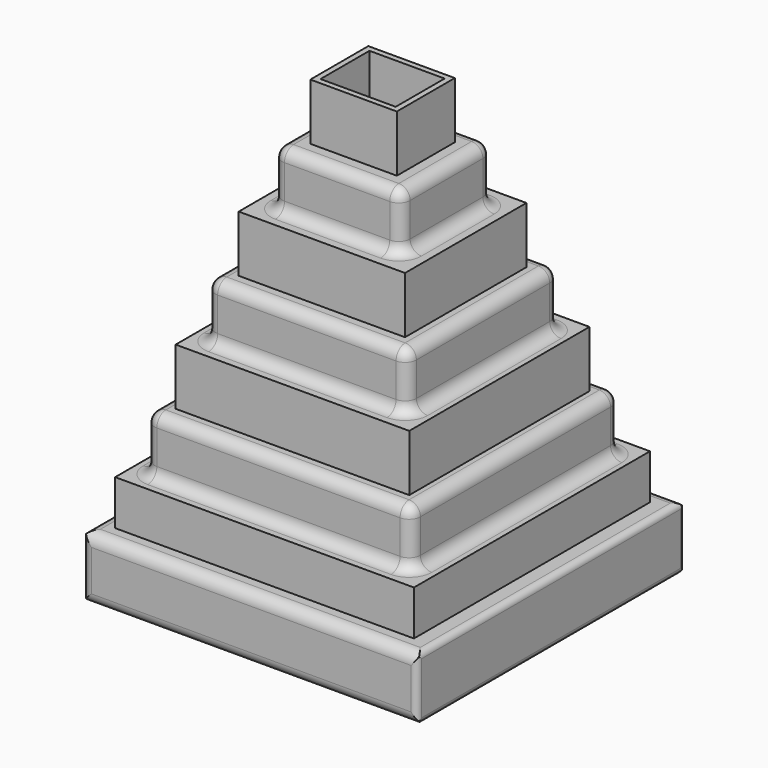
from build123d import *

# Parameters (mm, degrees)
F0_W         = 151.3316631317
F0_H         = 150.4956334829
F1_DEPTH     = 28.5412985831
F2_W         = 134.191930294
F2_H         = 132.5197666883
F3_DEPTH     = 20.1653186232
F4_W         = 119.4145902991
F4_H         = 116.9039234519
F5_DEPTH     = 25.4
F6_W         = 104.9288511276
F6_H         = 101.1665165424
F7_DEPTH     = 25.4
F8_W         = 90.2792215347
F8_H         = 84.9945694208
F9_DEPTH     = 25.4
F10_W        = 74.6954381466
F10_H        = 68.1595951319
F11_DEPTH    = 25.4
F12_W        = 57.4390292168
F12_H        = 51.001906395
F13_DEPTH    = 25.4
F14_W        = 38.8528704643
F14_H        = 32.552421093
F15_DEPTH    = 25.4
F16_T        = -2.54
F17_R        = 2.5998669894
F18_T1_DEPTH = 174.1317961423
F18_T3_DEPTH = 53.9412985831
F19_T1_DEPTH = 170.815633483
F19_T3_DEPTH = 53.9412985831
F20_T1_DEPTH = 169.0517961423
F21_R        = 5.08


# Not quite as in the source:
# - a fillet or chamfer that OpenCascade refuses, or shapes differently, is made with other operations: its cross-section is extruded or revolved along the edge and cut away or added


with BuildPart() as f1:
    # F0 (on Top) → F1 (new body)
    with BuildSketch(Plane.XY):
        Rectangle(F0_W, F0_H)
    extrude(amount=F1_DEPTH)

    # F2 (on face) → F3 (join)
    with BuildSketch(Plane.XY.offset(28.5412985831)):
        Rectangle(F2_W, F2_H)
    extrude(amount=F3_DEPTH)

    # F4 (on face) → F5 (join)
    with BuildSketch(Plane.XY.offset(48.7066172063)):
        Rectangle(F4_W, F4_H)
    extrude(amount=F5_DEPTH)

    # F6 (on face) → F7 (join)
    with BuildSketch(Plane.XY.offset(74.1066172063)):
        Rectangle(F6_W, F6_H)
    extrude(amount=F7_DEPTH)

    # F8 (on face) → F9 (join)
    with BuildSketch(Plane.XY.offset(99.5066172063)):
        Rectangle(F8_W, F8_H)
    extrude(amount=F9_DEPTH)

    # F10 (on face) → F11 (join)
    with BuildSketch(Plane.XY.offset(124.9066172063)):
        Rectangle(F10_W, F10_H)
    extrude(amount=F11_DEPTH)

    # F12 (on face) → F13 (join)
    with BuildSketch(Plane.XY.offset(150.3066172063)):
        Rectangle(F12_W, F12_H)
    extrude(amount=F13_DEPTH)

    # F14 (on face) → F15 (join)
    with BuildSketch(Plane.XY.offset(175.7066172063)):
        Rectangle(F14_W, F14_H)
    extrude(amount=F15_DEPTH)

    # F16
    f16_openings = [f1.faces().sort_by_distance(p)[0] for p in [
        (0, 0, 201.106617),
    ]]
    offset(amount=F16_T, openings=f16_openings, kind=Kind.INTERSECTION)

    # F17
    f17_edges = [f1.edges().sort_by_distance(p)[0] for p in [
        (75.665832, -75.247817, 14.270649),
        (75.665832, 75.247817, 14.270649),
        (75.665832, 0, 0),
        (75.665832, 0, 28.541299),
    ]]
    fillet(f17_edges, radius=F17_R)

    # F18: fillet of radius 5.08 on 4 edges, made by hand

    # F18_s2 → F18_t1 (cut)
    with BuildSketch(Plane.YZ.offset(-88.3658315659)):
        with BuildLine():
            ThreePointArc((-75.2478167415, 5.08), (-73.7599191899, 1.4878975516), (-70.1678167415, 0))
            Line((-70.1678167415, 0), (-75.2478167415, 0))
            Line((-75.2478167415, 0), (-75.2478167415, 5.08))
        make_face()
        with BuildLine():
            ThreePointArc((-75.2478167415, 23.4612985831), (-73.7599191899, 27.0534010316), (-70.1678167415, 28.5412985831))
            Line((-70.1678167415, 28.5412985831), (-75.2478167415, 28.5412985831))
            Line((-75.2478167415, 28.5412985831), (-75.2478167415, 23.4612985831))
        make_face()
    extrude(amount=F18_T1_DEPTH, mode=Mode.SUBTRACT)

    # F18_s4 → F18_t3 (cut)
    with BuildSketch(Plane.XY.offset(-12.7)):
        with BuildLine():
            ThreePointArc((-70.5858315659, -75.2478167415), (-74.1779340143, -73.7599191899), (-75.6658315659, -70.1678167415))
            Line((-75.6658315659, -70.1678167415), (-75.6658315659, -75.2478167415))
            Line((-75.6658315659, -75.2478167415), (-70.5858315659, -75.2478167415))
        make_face()
    extrude(amount=F18_T3_DEPTH, mode=Mode.SUBTRACT)

    # F19: fillet of radius 5.08 on 4 edges, made by hand

    # F19_s2 → F19_t1 (cut)
    with BuildSketch(Plane.XZ.offset(-87.9478167415)):
        with BuildLine():
            ThreePointArc((-70.5858315659, 0), (-74.1779340143, 1.4878975516), (-75.6658315659, 5.08))
            Line((-75.6658315659, 5.08), (-75.6658315659, 0))
            Line((-75.6658315659, 0), (-70.5858315659, 0))
        make_face()
        with BuildLine():
            ThreePointArc((-70.5858315659, 28.5412985831), (-74.1779340143, 27.0534010316), (-75.6658315659, 23.4612985831))
            Line((-75.6658315659, 23.4612985831), (-75.6658315659, 28.5412985831))
            Line((-75.6658315659, 28.5412985831), (-70.5858315659, 28.5412985831))
        make_face()
    extrude(amount=F19_T1_DEPTH, mode=Mode.SUBTRACT)

    # F19_s4 → F19_t3 (cut)
    with BuildSketch(Plane.XY.offset(-12.7)):
        with BuildLine():
            ThreePointArc((-70.5858315659, 75.2478167415), (-74.1779340143, 73.7599191899), (-75.6658315659, 70.1678167415))
            Line((-75.6658315659, 70.1678167415), (-75.6658315659, 75.2478167415))
            Line((-75.6658315659, 75.2478167415), (-70.5858315659, 75.2478167415))
        make_face()
    extrude(amount=F19_T3_DEPTH, mode=Mode.SUBTRACT)

    # F20: fillet of radius 5.08 on 4 edges, made by hand

    # F20_s2 → F20_t1 (cut)
    with BuildSketch(Plane.YZ.offset(-83.2858315659)):
        with BuildLine():
            ThreePointArc((70.1678167415, 0), (73.7599191899, 1.4878975516), (75.2478167415, 5.08))
            Line((75.2478167415, 5.08), (75.2478167415, 0))
            Line((75.2478167415, 0), (70.1678167415, 0))
        make_face()
        with BuildLine():
            ThreePointArc((70.1678167415, 28.5412985831), (73.7599191899, 27.0534010316), (75.2478167415, 23.4612985831))
            Line((75.2478167415, 23.4612985831), (75.2478167415, 28.5412985831))
            Line((75.2478167415, 28.5412985831), (70.1678167415, 28.5412985831))
        make_face()
    extrude(amount=F20_T1_DEPTH, mode=Mode.SUBTRACT)

    # F21
    f21_edges = [f1.edges().sort_by_distance(p)[0] for p in [
        (59.707295, 58.451962, 61.406617),
        (-59.707295, 58.451962, 61.406617),
        (0, 58.451962, 48.706617),
        (0, 58.451962, 74.106617),
        (45.139611, 42.497285, 112.206617),
        (-45.139611, 42.497285, 112.206617),
        (0, 42.497285, 99.506617),
        (0, 42.497285, 124.906617),
        (28.719515, 25.500953, 163.006617),
        (-28.719515, 25.500953, 163.006617),
        (0, 25.500953, 150.306617),
        (0, 25.500953, 175.706617),
        (59.707295, -58.451962, 61.406617),
        (59.707295, 0, 48.706617),
        (59.707295, 0, 74.106617),
        (45.139611, -42.497285, 112.206617),
        (45.139611, 0, 99.506617),
        (45.139611, 0, 124.906617),
        (28.719515, -25.500953, 163.006617),
        (28.719515, 0, 150.306617),
        (28.719515, 0, 175.706617),
        (-28.719515, -25.500953, 163.006617),
        (-28.719515, 0, 150.306617),
        (-28.719515, 0, 175.706617),
        (-45.139611, -42.497285, 112.206617),
        (-45.139611, 0, 99.506617),
        (-45.139611, 0, 124.906617),
        (-59.707295, -58.451962, 61.406617),
        (-59.707295, 0, 48.706617),
        (-59.707295, 0, 74.106617),
        (0, -58.451962, 48.706617),
        (0, -58.451962, 74.106617),
        (0, -42.497285, 99.506617),
        (0, -42.497285, 124.906617),
        (0, -25.500953, 150.306617),
        (0, -25.500953, 175.706617),
    ]]
    fillet(f21_edges, radius=F21_R)


solid = f1.part
